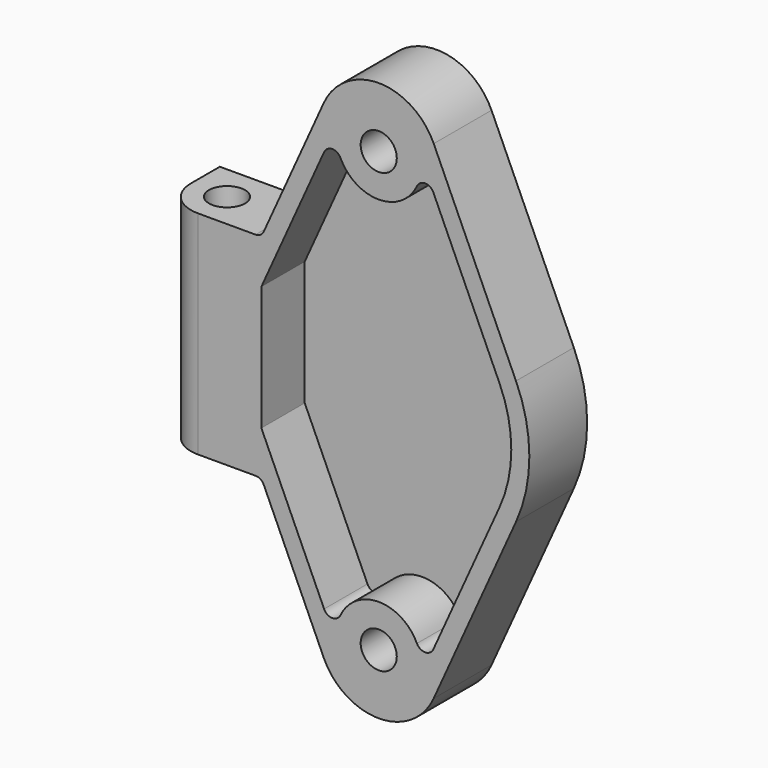
from build123d import *

# Parameters (mm, degrees)
F0_R     = 2
F1_DEPTH = 8
F2_DEPTH = 2
F3_R     = 1
F5_D     = 4
F6_R     = 4


# Not quite as in the source:
# - a feature names something its author has since deleted; it is built from what else it names


with BuildPart() as f1:
    # F0 (on Front) → F1 (new body)
    with BuildSketch(Plane.XZ):
        with BuildLine():
            Line((15.1970139668, 6.8636525628), (6.0880650012, 27.0320429916))
            ThreePointArc((6.0880650012, 27.0320429916), (0, 30.9626), (-6.0880650012, 27.0320429916))
            Line((-6.0880650012, 27.0320429916), (-12.9901204821, 11.75))
            Line((-12.9901204821, 11.75), (-12.9901204821, 6.8910419314))
            Line((-12.9901204821, 6.8910419314), (-6.0462846285, 22.2655920687))
            ThreePointArc((-6.0462846285, 22.2655920687), (-5.1436901116, 22.8539427752), (-4.2309206889, 22.2815046593))
            ThreePointArc((-4.2309206889, 22.2815046593), (0, 19.6022), (4.2309206889, 22.2815046593))
            ThreePointArc((4.2309206889, 22.2815046593), (5.1436901116, 22.8539427752), (6.0462846285, 22.2655920687))
            Line((6.0462846285, 22.2655920687), (13.3742945868, 6.0404308054))
            ThreePointArc((13.3742945868, 6.0404308054), (14.6751, 0), (13.3742945868, -6.0404308054))
            Line((13.3742945868, -6.0404308054), (6.0462846285, -22.2655920687))
            ThreePointArc((6.0462846285, -22.2655920687), (5.1436901116, -22.8539427752), (4.2309206889, -22.2815046593))
            ThreePointArc((4.2309206889, -22.2815046593), (0, -19.6022), (-4.2309206889, -22.2815046593))
            ThreePointArc((-4.2309206889, -22.2815046593), (-5.1436901116, -22.8539427752), (-6.0462846285, -22.2655920687))
            Line((-6.0462846285, -22.2655920687), (-12.9901204821, -6.8910419314))
            Line((-12.9901204821, -6.8910419314), (-12.9901204821, -11.75))
            Line((-12.9901204821, -11.75), (-6.0880650012, -27.0320429916))
            ThreePointArc((-6.0880650012, -27.0320429916), (0, -30.9626), (6.0880650012, -27.0320429916))
            Line((6.0880650012, -27.0320429916), (15.1970139668, -6.8636525628))
            ThreePointArc((15.1970139668, -6.8636525628), (16.6751, 0), (15.1970139668, 6.8636525628))
        make_face()
        with Locations((0, -24.2824)):
            Circle(F0_R, mode=Mode.SUBTRACT)
        with Locations((0, 24.2824)):
            Circle(F0_R, mode=Mode.SUBTRACT)
        Polygon((-12.9901204821, 6.8910419314), (-12.9901204821, 11.75), (-23.9901204821, 11.75), (-23.9901204821, -11.75), (-12.9901204821, -11.75), (-12.9901204821, -6.8910419314), align=None)
    extrude(amount=F1_DEPTH)

    # F0 (on Front) → F2 (join)
    with BuildSketch(Plane.XZ):
        with BuildLine():
            Line((-6.0462846285, 22.2655920687), (-12.9901204821, 6.8910419314))
            Line((-12.9901204821, 6.8910419314), (-12.9901204821, -6.8910419314))
            Line((-12.9901204821, -6.8910419314), (-6.0462846285, -22.2655920687))
            ThreePointArc((-6.0462846285, -22.2655920687), (-5.1436901116, -22.8539427752), (-4.2309206889, -22.2815046593))
            ThreePointArc((-4.2309206889, -22.2815046593), (0, -19.6022), (4.2309206889, -22.2815046593))
            ThreePointArc((4.2309206889, -22.2815046593), (5.1436901116, -22.8539427752), (6.0462846285, -22.2655920687))
            Line((6.0462846285, -22.2655920687), (13.3742945868, -6.0404308054))
            ThreePointArc((13.3742945868, -6.0404308054), (14.6751, 0), (13.3742945868, 6.0404308054))
            Line((13.3742945868, 6.0404308054), (6.0462846285, 22.2655920687))
            ThreePointArc((6.0462846285, 22.2655920687), (5.1436901116, 22.8539427752), (4.2309206889, 22.2815046593))
            ThreePointArc((4.2309206889, 22.2815046593), (0, 19.6022), (-4.2309206889, 22.2815046593))
            ThreePointArc((-4.2309206889, 22.2815046593), (-5.1436901116, 22.8539427752), (-6.0462846285, 22.2655920687))
        make_face()
        Polygon((-12.9901204821, 6.8910419314), (-12.9901204821, 11.75), (-23.9901204821, 11.75), (-23.9901204821, -11.75), (-12.9901204821, -11.75), (-12.9901204821, -6.8910419314), align=None)
        with BuildLine():
            Line((15.1970139668, 6.8636525628), (6.0880650012, 27.0320429916))
            ThreePointArc((6.0880650012, 27.0320429916), (0, 30.9626), (-6.0880650012, 27.0320429916))
            Line((-6.0880650012, 27.0320429916), (-12.9901204821, 11.75))
            Line((-12.9901204821, 11.75), (-12.9901204821, 6.8910419314))
            Line((-12.9901204821, 6.8910419314), (-6.0462846285, 22.2655920687))
            ThreePointArc((-6.0462846285, 22.2655920687), (-5.1436901116, 22.8539427752), (-4.2309206889, 22.2815046593))
            ThreePointArc((-4.2309206889, 22.2815046593), (0, 19.6022), (4.2309206889, 22.2815046593))
            ThreePointArc((4.2309206889, 22.2815046593), (5.1436901116, 22.8539427752), (6.0462846285, 22.2655920687))
            Line((6.0462846285, 22.2655920687), (13.3742945868, 6.0404308054))
            ThreePointArc((13.3742945868, 6.0404308054), (14.6751, 0), (13.3742945868, -6.0404308054))
            Line((13.3742945868, -6.0404308054), (6.0462846285, -22.2655920687))
            ThreePointArc((6.0462846285, -22.2655920687), (5.1436901116, -22.8539427752), (4.2309206889, -22.2815046593))
            ThreePointArc((4.2309206889, -22.2815046593), (0, -19.6022), (-4.2309206889, -22.2815046593))
            ThreePointArc((-4.2309206889, -22.2815046593), (-5.1436901116, -22.8539427752), (-6.0462846285, -22.2655920687))
            Line((-6.0462846285, -22.2655920687), (-12.9901204821, -6.8910419314))
            Line((-12.9901204821, -6.8910419314), (-12.9901204821, -11.75))
            Line((-12.9901204821, -11.75), (-6.0880650012, -27.0320429916))
            ThreePointArc((-6.0880650012, -27.0320429916), (0, -30.9626), (6.0880650012, -27.0320429916))
            Line((6.0880650012, -27.0320429916), (15.1970139668, -6.8636525628))
            ThreePointArc((15.1970139668, -6.8636525628), (16.6751, 0), (15.1970139668, 6.8636525628))
        make_face()
        with Locations((0, -24.2824)):
            Circle(F0_R, mode=Mode.SUBTRACT)
        with Locations((0, 24.2824)):
            Circle(F0_R, mode=Mode.SUBTRACT)
    extrude(amount=F2_DEPTH)

    # F3
    f3_edges = [f1.edges().sort_by_distance(p)[0] for p in [
        (-12.99012, -4, -11.75),
        (-12.99012, -4, 11.75),
    ]]
    fillet(f3_edges, radius=F3_R)

    # F5 (through all)
    with Locations(Plane.XY.offset(11.75)):
        with Locations((-19.9901204821, -4)):
            Hole(F5_D / 2)

    # F6
    f6_edges = [f1.edges().sort_by_distance(p)[0] for p in [
        (-23.99012, -8, 0),
    ]]
    fillet(f6_edges, radius=F6_R)


solid = f1.part
